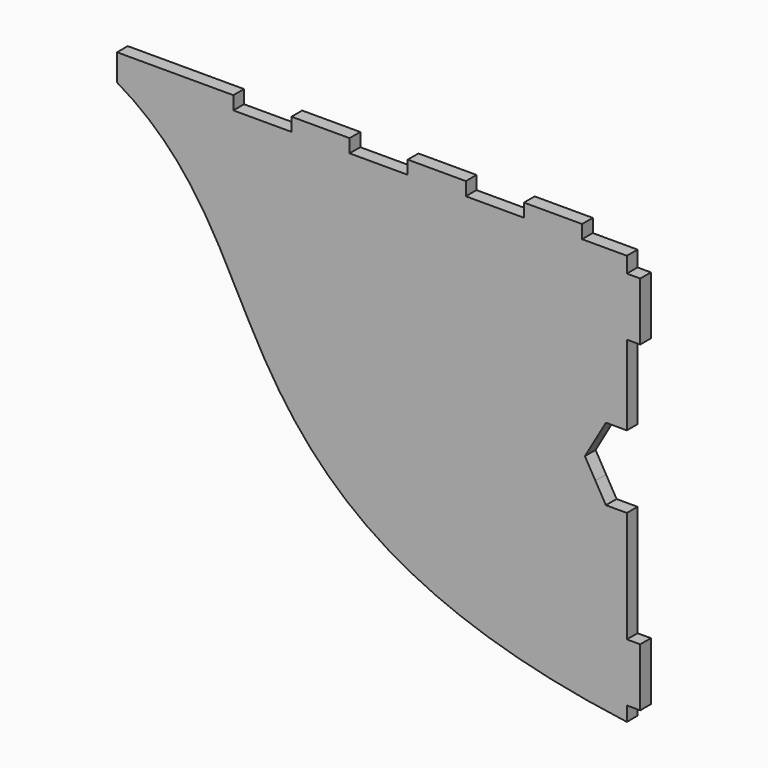
from build123d import *

# Parameters (mm, degrees)
F0_W      = 279.4
F0_H      = 330.2
F1_DEPTH  = 5.842
F2_W      = 25.4
F2_H      = 5.842
F2_W_2    = 76.2
F2_W_3    = 5.842
F2_H_2    = 25.4
F2_H_3    = 38.1
F3_DEPTH  = 5.842
F5_W      = 5.842
F5_H      = 12.7
F6_DEPTH  = 5.842
F7_DEPTH  = 5.842
F8_W      = 5.842
F8_H      = 48.641
F8_H_2    = 34.925
F8_H_3    = 11.684
F9_DEPTH  = 5.842
F10_W     = 246.7240431406
F10_H     = 1.016
F11_DEPTH = 5.842
F12_W     = 25.4
F12_H     = 5.842
F12_W_2   = 19.558
F13_DEPTH = 5.842


with BuildPart() as f1:
    # F0 (on Front) → F1 (new body)
    with BuildSketch(Plane.XZ):
        with Locations((25.751306051, 40.8756073241)):
            Rectangle(F0_W, F0_H)
    extrude(amount=F1_DEPTH)

    # F2 (on face) → F3 (cut, through all)
    with BuildSketch(Plane.XZ.offset(5.842)):
        with Locations((152.751306051, -121.3033926759)):
            Rectangle(F2_W, F2_H)
        with Locations((101.951306051, -121.3033926759)):
            Rectangle(F2_W, F2_H)
        with Locations((51.151306051, -121.3033926759)):
            Rectangle(F2_W, F2_H)
        with Locations((0.351306051, -121.3033926759)):
            Rectangle(F2_W, F2_H)
        with Locations((-75.848693949, -121.3033926759)):
            Rectangle(F2_W_2, F2_H)
        with Locations((162.530306051, -86.1243926759)):
            Rectangle(F2_W_3, F2_H_2)
        with Locations((162.530306051, -28.9743926759)):
            Rectangle(F2_W_3, F2_H_3)
        with Locations((-111.027693949, -86.1243926759)):
            Rectangle(F2_W_3, F2_H_2)
        with Locations((-111.027693949, -35.3243926759)):
            Rectangle(F2_W_3, F2_H_2)
        with Locations((-111.027693949, 15.4756073241)):
            Rectangle(F2_W_3, F2_H_2)
        with Locations((-111.027693949, 66.2756073241)):
            Rectangle(F2_W_3, F2_H_2)
        with Locations((-111.027693949, 167.8756073241)):
            Rectangle(F2_W_3, F2_H_2)
        with Locations((-111.027693949, 117.0756073241)):
            Rectangle(F2_W_3, F2_H_2)
    extrude(amount=-F3_DEPTH, mode=Mode.SUBTRACT)

    # F5 (on face) → F6 (cut, through all)
    with BuildSketch(Plane.XZ.offset(5.842)):
        with Locations((162.530306051, 2.7756073241)):
            Rectangle(F5_W, F5_H)
    extrude(amount=-F6_DEPTH, mode=Mode.SUBTRACT)

    # F4 (on face) → F7 (cut, through all)
    with BuildSketch(Plane.XZ.offset(5.842)):
        with BuildLine():
            Line((165.451306051, 15.4756073241), (159.609306051, 15.4756073241))
            add(Edge.make_bspline(
                [(159.609306051, 15.4756073241), (73.376306051, 28.1756073241), (-24.3765935073, 60.3637718481), (-21.873693949, 193.2756073241), (-113.948693949, 205.9756073241)],
                knots=[0, 0, 0, 0, 0.507272, 1, 1, 1, 1], degree=3))
            Line((-113.948693949, 205.9756073241), (-113.948693949, 180.5756073241))
            Line((-113.948693949, 180.5756073241), (-108.106693949, 180.5756073241))
            Line((-108.106693949, 180.5756073241), (-108.106693949, 155.1756073241))
            Line((-108.106693949, 155.1756073241), (-113.948693949, 155.1756073241))
            Line((-113.948693949, 155.1756073241), (-113.948693949, 129.7756073241))
            Line((-113.948693949, 129.7756073241), (-108.106693949, 129.7756073241))
            Line((-108.106693949, 129.7756073241), (-108.106693949, 104.3756073241))
            Line((-108.106693949, 104.3756073241), (-113.948693949, 104.3756073241))
            Line((-113.948693949, 104.3756073241), (-113.948693949, 78.9756073241))
            Line((-113.948693949, 78.9756073241), (-108.106693949, 78.9756073241))
            Line((-108.106693949, 78.9756073241), (-108.106693949, 53.5756073241))
            Line((-108.106693949, 53.5756073241), (-113.948693949, 53.5756073241))
            Line((-113.948693949, 53.5756073241), (-113.948693949, 28.1756073241))
            Line((-113.948693949, 28.1756073241), (-108.106693949, 28.1756073241))
            Line((-108.106693949, 28.1756073241), (-108.106693949, 2.7756073241))
            Line((-108.106693949, 2.7756073241), (-113.948693949, 2.7756073241))
            Line((-113.948693949, 2.7756073241), (-113.948693949, -22.6243926759))
            Line((-113.948693949, -22.6243926759), (-108.106693949, -22.6243926759))
            Line((-108.106693949, -22.6243926759), (-108.106693949, -48.0243926759))
            Line((-108.106693949, -48.0243926759), (-113.948693949, -48.0243926759))
            Line((-113.948693949, -48.0243926759), (-113.948693949, -73.4243926759))
            Line((-113.948693949, -73.4243926759), (-108.106693949, -73.4243926759))
            Line((-108.106693949, -73.4243926759), (-108.106693949, -98.8243926759))
            Line((-108.106693949, -98.8243926759), (-113.948693949, -98.8243926759))
            Line((-113.948693949, -98.8243926759), (-113.948693949, -118.3823926759))
            Line((-113.948693949, -118.3823926759), (-37.748693949, -118.3823926759))
            Line((-37.748693949, -118.3823926759), (-37.748693949, -124.2243926759))
            Line((-37.748693949, -124.2243926759), (-12.348693949, -124.2243926759))
            Line((-12.348693949, -124.2243926759), (-12.348693949, -118.3823926759))
            Line((-12.348693949, -118.3823926759), (13.051306051, -118.3823926759))
            Line((13.051306051, -118.3823926759), (13.051306051, -124.2243926759))
            Line((13.051306051, -124.2243926759), (38.451306051, -124.2243926759))
            Line((38.451306051, -124.2243926759), (38.451306051, -118.3823926759))
            Line((38.451306051, -118.3823926759), (63.851306051, -118.3823926759))
            Line((63.851306051, -118.3823926759), (63.851306051, -124.2243926759))
            Line((63.851306051, -124.2243926759), (89.251306051, -124.2243926759))
            Line((89.251306051, -124.2243926759), (89.251306051, -118.3823926759))
            Line((89.251306051, -118.3823926759), (114.651306051, -118.3823926759))
            Line((114.651306051, -118.3823926759), (114.651306051, -124.2243926759))
            Line((114.651306051, -124.2243926759), (140.051306051, -124.2243926759))
            Line((140.051306051, -124.2243926759), (140.051306051, -118.3823926759))
            Line((140.051306051, -118.3823926759), (165.451306051, -118.3823926759))
            Line((165.451306051, -118.3823926759), (165.451306051, -98.8243926759))
            Line((165.451306051, -98.8243926759), (159.609306051, -98.8243926759))
            Line((159.609306051, -98.8243926759), (159.609306051, -73.4243926759))
            Line((159.609306051, -73.4243926759), (165.451306051, -73.4243926759))
            Line((165.451306051, -73.4243926759), (165.451306051, -48.0243926759))
            Line((165.451306051, -48.0243926759), (159.609306051, -48.0243926759))
            Line((159.609306051, -48.0243926759), (159.609306051, -9.9243926759))
            Line((159.609306051, -9.9243926759), (165.451306051, -9.9243926759))
            Line((165.451306051, -9.9243926759), (165.451306051, 15.4756073241))
        make_face()
        with BuildLine():
            add(Edge.make_bspline(
                [(159.609306051, 15.4756073241), (73.376306051, 28.1756073241), (-24.3765935073, 60.3637718481), (-21.873693949, 193.2756073241), (-113.948693949, 205.9756073241)],
                knots=[0, 0, 0, 0, 0.507272, 1, 1, 1, 1], degree=3))
            Line((159.609306051, 15.4756073241), (159.609306051, 21.8256073241))
            add(Edge.make_bspline(
                [(159.609306051, 21.8256073241), (63.851306051, 34.5256073241), (-5.6173037023, 95.4914607938), (-31.4644745687, 187.7697107475), (-87.114737086, 205.9756073241)],
                knots=[0, 0, 0, 0, 0.5236819738, 0.940243193, 0.940243193, 0.940243193, 0.940243193], degree=3))
            Line((-87.114737086, 205.9756073241), (-113.948693949, 205.9756073241))
        make_face()
    extrude(amount=-F7_DEPTH, mode=Mode.SUBTRACT)

    # F8 (on face) → F9 (cut, through all)
    with BuildSketch(Plane.XZ.offset(5.842)):
        Polygon((165.451306051, 15.4756073241), (165.451306051, 28.1756073241), (159.609306051, 28.1756073241), (159.609306051, 21.8256073241), (159.609306051, 15.4756073241), align=None)
        with Locations((162.530306051, 77.8961073241)):
            Rectangle(F8_W, F8_H)
        with BuildLine():
            Line((159.609306051, 102.2166073241), (165.451306051, 102.2166073241))
            Line((165.451306051, 102.2166073241), (165.451306051, 103.3306229057))
            ThreePointArc((165.451306051, 103.3306229057), (162.5829399691, 102.4975980153), (159.609306051, 102.2166073241))
        make_face()
        with BuildLine():
            ThreePointArc((145.861152343, 110.1541080567), (151.6718056847, 104.3434542505), (159.609306051, 102.2166073241))
            Line((159.609306051, 102.2166073241), (159.609306051, 133.9666073241))
            ThreePointArc((159.609306051, 133.9666073241), (151.6718056847, 131.8397603977), (145.861152343, 126.0291065915))
            ThreePointArc((145.861152343, 126.0291065915), (143.734306051, 118.0916073241), (145.861152343, 110.1541080567))
        make_face()
        with BuildLine():
            Line((150.4438705276, 102.2166073241), (159.609306051, 102.2166073241))
            ThreePointArc((159.609306051, 102.2166073241), (151.6718056847, 104.3434542505), (145.861152343, 110.1541080567))
            Line((145.861152343, 110.1541080567), (150.4438705276, 102.2166073241))
        make_face()
        with BuildLine():
            Line((159.609306051, 133.9666073241), (159.609306051, 102.2166073241))
            ThreePointArc((159.609306051, 102.2166073241), (162.5829399691, 102.4975980153), (165.451306051, 103.3306229057))
            Line((165.451306051, 103.3306229057), (165.451306051, 132.8525917425))
            ThreePointArc((165.451306051, 132.8525917425), (162.5829399691, 133.6856166328), (159.609306051, 133.9666073241))
        make_face()
        with BuildLine():
            Line((165.451306051, 133.9666073241), (159.609306051, 133.9666073241))
            ThreePointArc((159.609306051, 133.9666073241), (162.5829399691, 133.6856166328), (165.451306051, 132.8525917425))
            Line((165.451306051, 132.8525917425), (165.451306051, 133.9666073241))
        make_face()
        with BuildLine():
            ThreePointArc((145.861152343, 126.0291065915), (151.6718056847, 131.8397603977), (159.609306051, 133.9666073241))
            Line((159.609306051, 133.9666073241), (150.4438705276, 133.9666073241))
            Line((150.4438705276, 133.9666073241), (145.861152343, 126.0291065915))
        make_face()
        with Locations((162.530306051, 151.4291073241)):
            Rectangle(F8_W, F8_H_2)
        with BuildLine():
            Line((141.2784350042, 118.0916073241), (145.861152343, 110.1541080567))
            ThreePointArc((145.861152343, 110.1541080567), (143.734306051, 118.0916073241), (145.861152343, 126.0291065915))
            Line((145.861152343, 126.0291065915), (141.2784350042, 118.0916073241))
        make_face()
        with Locations((162.530306051, 200.1336073241)):
            Rectangle(F8_W, F8_H_3)
    extrude(amount=-F9_DEPTH, mode=Mode.SUBTRACT)

    # F10 (on face) → F11 (join, through all)
    with BuildSketch(Plane.XZ.offset(5.842)):
        with Locations((36.2472844807, 206.4836073241)):
            Rectangle(F10_W, F10_H)
    extrude(amount=-F11_DEPTH)

    # F12 (on face) → F13 (cut, through all)
    with BuildSketch(Plane.XZ.offset(5.842)):
        with Locations((51.151306051, 204.0706073241)):
            Rectangle(F12_W, F12_H)
        with Locations((101.951306051, 204.0706073241)):
            Rectangle(F12_W, F12_H)
        with Locations((149.830306051, 204.0706073241)):
            Rectangle(F12_W_2, F12_H)
        with BuildLine():
            add(Edge.make_bspline(
                [(-64.0656111495, 195.8912068503), (-64.4986133811, 197.8821506555), (-64.5462177809, 200.9608220943), (-64.8897370896, 206.9916073241)],
                knots=[0.7783755915, 0.7783755915, 0.7783755915, 0.7783755915, 1, 1, 1, 1], degree=3))
            Line((-64.8897370896, 206.9916073241), (-87.1147370896, 206.9916073241))
            Line((-87.1147370896, 206.9916073241), (-87.1147370896, 205.9756073241))
            add(Edge.make_bspline(
                [(-64.0656111419, 195.8912068549), (-70.8038372609, 199.7329606353), (-78.4197996839, 203.1310721158), (-87.114737086, 205.9756073241)],
                knots=[0.8751586172, 0.8751586172, 0.8751586172, 0.8751586172, 0.940243193, 0.940243193, 0.940243193, 0.940243193], degree=3))
        make_face()
        with Locations((0.351306051, 204.0706073241)):
            Rectangle(F12_W, F12_H)
        with BuildLine():
            Line((-63.148693949, 195.362557311), (-63.148693949, 206.9916073241))
            Line((-63.148693949, 206.9916073241), (-64.8897370896, 206.9916073241))
            add(Edge.make_bspline(
                [(-64.0656111495, 195.8912068503), (-64.4986133811, 197.8821506555), (-64.5462177809, 200.9608220943), (-64.8897370896, 206.9916073241)],
                knots=[0.7783755915, 0.7783755915, 0.7783755915, 0.7783755915, 1, 1, 1, 1], degree=3))
            add(Edge.make_bspline(
                [(-63.148693949, 195.362557311), (-63.4525182871, 195.5396905387), (-63.7581509788, 195.7159105346), (-64.0656111419, 195.8912068549)],
                knots=[0.8721888572, 0.8721888572, 0.8721888572, 0.8721888572, 0.8751586172, 0.8751586172, 0.8751586172, 0.8751586172], degree=3))
        make_face()
    extrude(amount=-F13_DEPTH, mode=Mode.SUBTRACT)


solid = f1.part
